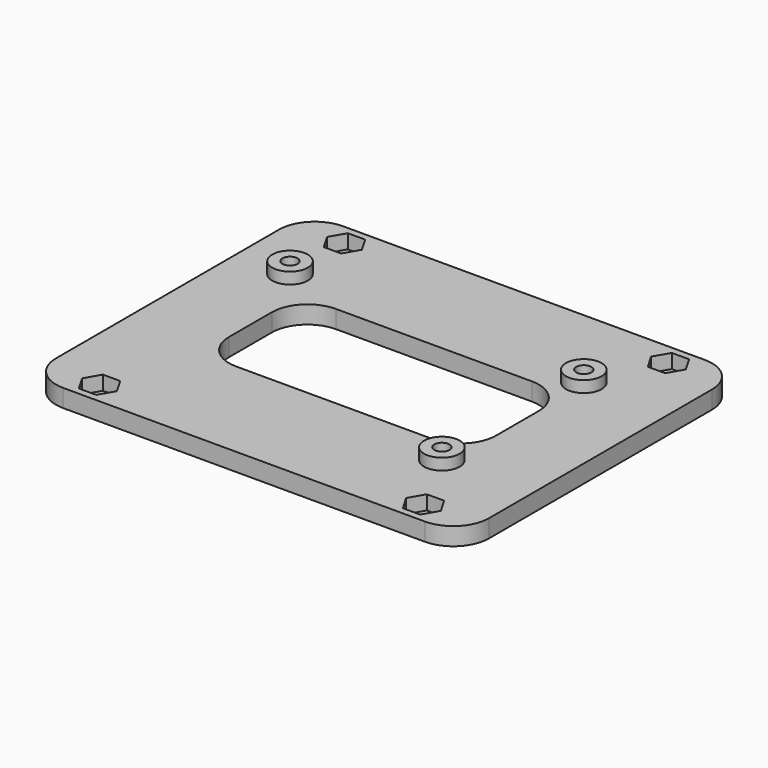
from build123d import *

# Parameters (mm, degrees)
F0_W         = 121.6
F0_H         = 78.3
F0_R         = 2.125
F1_DEPTH     = 5
F2_R         = 5
F2_R_2       = 2.125
F3_DEPTH     = 3.2
F5_DEPTH     = 4
F6_W         = 121.6
F6_H         = 10
F6_R         = 2.25
F7_DEPTH     = 5
F8_R         = 10
F9_T3_DEPTH  = 9.8067065447
F9_S4_R      = 2.125
F9_T5_DEPTH  = 7
F9_T8_DEPTH  = 9.8067065447
F9_S9_R      = 2.125
F9_T10_DEPTH = 6
F9_T13_DEPTH = 9.8067065447
F9_S14_R     = 2.125
F9_T15_DEPTH = 7
F9_T18_DEPTH = 9.8067065447
F9_S19_R     = 2.125
F9_T20_DEPTH = 7
F9_T23_DEPTH = 9.8067065447
F9_S24_R     = 2.125
F9_T25_DEPTH = 7
F9_T28_DEPTH = 9.8067065447
F9_S29_R     = 2.125
F9_T30_DEPTH = 6
F9_T33_DEPTH = 9.8067065447
F9_S34_R     = 2.125
F9_T35_DEPTH = 6
F9_T38_DEPTH = 9.8067065447
F9_S39_R     = 2.125
F9_T40_DEPTH = 7
F9_T43_DEPTH = 9.8067065447
F9_S44_R     = 2.125
F9_T45_DEPTH = 7
F9_T48_DEPTH = 9.8067065447
F9_S49_R     = 2.125
F9_T50_DEPTH = 7
F9_T53_DEPTH = 9.8067065447
F9_S54_R     = 2.125
F9_T55_DEPTH = 7
F9_T58_DEPTH = 9.8067065447
F9_S59_R     = 2.125
F9_T60_DEPTH = 6
F9_T63_DEPTH = 9.8067065447
F9_S64_R     = 2.125
F9_T65_DEPTH = 7
F9_T68_DEPTH = 9.8067065447
F9_S69_R     = 2.125
F9_T70_DEPTH = 6
F9_T73_DEPTH = 9.8067065447
F9_S74_R     = 2.125
F9_T75_DEPTH = 7
F9_T78_DEPTH = 9.8067065447
F9_S79_R     = 2.125
F9_T80_DEPTH = 7
F9_T83_DEPTH = 9.8067065447
F9_S84_R     = 2.125
F9_T85_DEPTH = 6
F9_T88_DEPTH = 9.8067065447
F9_S89_R     = 2.125
F9_T90_DEPTH = 7
F11_DEPTH    = 4


# Not quite as in the source:
# - a fillet or chamfer that OpenCascade refuses, or shapes differently, is made with other operations: its cross-section is extruded or revolved along the edge and cut away or added


with BuildPart() as f1:
    # F0 (on Top) → F1 (new body)
    with BuildSketch(Plane.XY):
        Rectangle(F0_W, F0_H)
        with Locations((35.5, -24.05)):
            Circle(F0_R, mode=Mode.SUBTRACT)
        with BuildLine():
            ThreePointArc((37.5, -7.5), (34.5710678119, -14.5710678119), (27.5, -17.5))
            Line((27.5, -17.5), (-27.5, -17.5))
            ThreePointArc((-27.5, -17.5), (-34.5710678119, -14.5710678119), (-37.5, -7.5))
            Line((-37.5, -7.5), (-37.5, 7.5))
            ThreePointArc((-37.5, 7.5), (-34.5710678119, 14.5710678119), (-27.5, 17.5))
            Line((-27.5, 17.5), (27.5, 17.5))
            ThreePointArc((27.5, 17.5), (34.5710678119, 14.5710678119), (37.5, 7.5))
            Line((37.5, 7.5), (37.5, -7.5))
        make_face(mode=Mode.SUBTRACT)
        with Locations((-45.72, 24.15)):
            Circle(F0_R, mode=Mode.SUBTRACT)
        with Locations((36.8, 24.15)):
            Circle(F0_R, mode=Mode.SUBTRACT)
    extrude(amount=F1_DEPTH)

    # F2 (on face) → F3 (join)
    with BuildSketch(Plane.XY.offset(5)):
        with Locations((-45.72, 24.15)):
            Circle(F2_R)
        with Locations((-45.72, 24.15)):
            Circle(F2_R_2, mode=Mode.SUBTRACT)
        with Locations((36.8, 24.15)):
            Circle(F2_R)
        with Locations((36.8, 24.15)):
            Circle(F2_R_2, mode=Mode.SUBTRACT)
        with Locations((35.5, -24.05)):
            Circle(F2_R)
        with Locations((35.5, -24.05)):
            Circle(F2_R_2, mode=Mode.SUBTRACT)
    extrude(amount=F3_DEPTH)

    # F4 (on face) → F5 (cut)
    with BuildSketch(Plane(origin=(0, 0, 0), x_dir=(1, 0, 0), z_dir=(0, 0, -1))):
        Polygon((-44.0312504626, -21.225), (-47.4087495374, -21.225), (-49.0974990748, -24.15), (-47.4087495374, -27.075), (-44.0312504626, -27.075), (-42.3425009252, -24.15), align=None)
        Polygon((38.4887495374, -21.225), (35.1112504626, -21.225), (33.4225009252, -24.15), (35.1112504626, -27.075), (38.4887495374, -27.075), (40.1774990748, -24.15), align=None)
        Polygon((33.8112504626, 21.125), (37.1887495374, 21.125), (38.8774990748, 24.05), (37.1887495374, 26.975), (33.8112504626, 26.975), (32.1225009252, 24.05), align=None)
    extrude(amount=-F5_DEPTH, mode=Mode.SUBTRACT)

    # F6 (on Top) → F7 (join)
    with BuildSketch(Plane.XY):
        with Locations((0, 44.15)):
            Rectangle(F6_W, F6_H)
        with Locations((-45.5, 43)):
            Circle(F6_R, mode=Mode.SUBTRACT)
        with Locations((45.5, 43)):
            Circle(F6_R, mode=Mode.SUBTRACT)
        with Locations((0, -44.15)):
            Rectangle(F6_W, F6_H)
        with Locations((-45.5, -43)):
            Circle(F6_R, mode=Mode.SUBTRACT)
        with Locations((45.5, -43)):
            Circle(F6_R, mode=Mode.SUBTRACT)
    extrude(amount=F7_DEPTH)

    # F8
    f8_edges = [f1.edges().sort_by_distance(p)[0] for p in [
        (-60.8, 49.15, 2.5),
        (60.8, 49.15, 2.5),
        (-60.8, -49.15, 2.5),
        (60.8, -49.15, 2.5),
    ]]
    fillet(f8_edges, radius=F8_R)

    # F9: chamfer of 1.25 on 18 edges, made by hand


with BuildPart() as f9_tool1:
    # F9_s2 → F9_t3 (new body)
    with BuildSketch(Plane(origin=(0.9127211557, 1.5808794147, 0), x_dir=(0, 0, 1), z_dir=(-0.5, -0.8660254038, 0))):
        Polygon((2.75, -45.6939018343), (4, -44.4439018343), (4, -45.6939018343), align=None)
    extrude(amount=F9_T3_DEPTH)

    # F9_s4 → F9_t5 (cut, symmetric)
    with BuildSketch(Plane.XY.offset(3.4)):
        with Locations((35.5, -24.05)):
            Circle(F9_S4_R)
    extrude(amount=F9_T5_DEPTH, both=True, mode=Mode.SUBTRACT)


with BuildPart() as f9_tool6:
    # F9_s7 → F9_t8 (new body)
    with BuildSketch(Plane.YZ.offset(40.4033532723)):
        Polygon((-26.975, 2.75), (-25.725, 4), (-26.975, 4), align=None)
    extrude(amount=-F9_T8_DEPTH)

    # F9_s9 → F9_t10 (cut, symmetric)
    with BuildSketch(Plane.XY.offset(3.4)):
        with Locations((35.5, -24.05)):
            Circle(F9_S9_R)
    extrude(amount=F9_T10_DEPTH, both=True, mode=Mode.SUBTRACT)


with BuildPart() as f9_tool11:
    # F9_s12 → F9_t13 (new body)
    with BuildSketch(Plane(origin=(21.7406321167, -37.6558794147, 0), x_dir=(0, 0, 1), z_dir=(-0.5, 0.8660254038, 0))):
        Polygon((2.75, 15.7939018343), (4, 17.0439018343), (4, 15.7939018343), align=None)
    extrude(amount=F9_T13_DEPTH)

    # F9_s14 → F9_t15 (cut, symmetric)
    with BuildSketch(Plane.XY.offset(3.4)):
        with Locations((35.5, -24.05)):
            Circle(F9_S14_R)
    extrude(amount=F9_T15_DEPTH, both=True, mode=Mode.SUBTRACT)


with BuildPart() as f9_tool16:
    # F9_s17 → F9_t18 (new body)
    with BuildSketch(Plane(origin=(-3.9906321167, -6.9119775804, 0), x_dir=(0, 0, 1), z_dir=(0.5, 0.8660254038, 0))):
        Polygon((2.75, 39.8439018343), (4, 41.0939018343), (4, 39.8439018343), align=None)
    extrude(amount=F9_T18_DEPTH)

    # F9_s19 → F9_t20 (cut, symmetric)
    with BuildSketch(Plane.XY.offset(3.4)):
        with Locations((35.5, -24.05)):
            Circle(F9_S19_R)
    extrude(amount=F9_T20_DEPTH, both=True, mode=Mode.SUBTRACT)


with BuildPart() as f9_tool21:
    # F9_s22 → F9_t23 (new body)
    with BuildSketch(Plane(origin=(16.8372788443, -29.1630224196, 0), x_dir=(0, 0, 1), z_dir=(0.5, -0.8660254038, 0))):
        Polygon((2.75, -21.6439018343), (4, -20.3939018343), (4, -21.6439018343), align=None)
    extrude(amount=F9_T23_DEPTH)

    # F9_s24 → F9_t25 (cut, symmetric)
    with BuildSketch(Plane.XY.offset(3.4)):
        with Locations((35.5, -24.05)):
            Circle(F9_S24_R)
    extrude(amount=F9_T25_DEPTH, both=True, mode=Mode.SUBTRACT)


with BuildPart() as f9_tool26:
    # F9_s27 → F9_t28 (new body)
    with BuildSketch(Plane.YZ.offset(30.5966467277)):
        Polygon((-21.125, 2.75), (-22.375, 4), (-21.125, 4), align=None)
    extrude(amount=F9_T28_DEPTH)

    # F9_s29 → F9_t30 (cut, symmetric)
    with BuildSketch(Plane.XY.offset(3.4)):
        with Locations((35.5, -24.05)):
            Circle(F9_S29_R)
    extrude(amount=F9_T30_DEPTH, both=True, mode=Mode.SUBTRACT)


with BuildPart() as f9_tool31:
    # F9_s32 → F9_t33 (new body)
    with BuildSketch(Plane.YZ.offset(41.7033532723)):
        Polygon((21.225, 2.75), (22.475, 4), (21.225, 4), align=None)
    extrude(amount=-F9_T33_DEPTH)

    # F9_s34 → F9_t35 (cut, symmetric)
    with BuildSketch(Plane.XY.offset(3.4)):
        with Locations((36.8, 24.15)):
            Circle(F9_S34_R)
    extrude(amount=F9_T35_DEPTH, both=True, mode=Mode.SUBTRACT)


with BuildPart() as f9_tool36:
    # F9_s37 → F9_t38 (new body)
    with BuildSketch(Plane(origin=(1.1944198855, -2.0687959272, 0), x_dir=(0, 0, 1), z_dir=(-0.5, 0.8660254038, 0))):
        Polygon((2.75, 41.0197348593), (4, 42.2697348593), (4, 41.0197348593), align=None)
    extrude(amount=F9_T38_DEPTH)

    # F9_s39 → F9_t40 (cut, symmetric)
    with BuildSketch(Plane.XY.offset(3.4)):
        with Locations((36.8, 24.15)):
            Circle(F9_S39_R)
    extrude(amount=F9_T40_DEPTH, both=True, mode=Mode.SUBTRACT)


with BuildPart() as f9_tool41:
    # F9_s42 → F9_t43 (new body)
    with BuildSketch(Plane(origin=(17.2055801145, 29.8009389321, 0), x_dir=(0, 0, 1), z_dir=(0.5, 0.8660254038, 0))):
        Polygon((2.75, 16.8697348593), (4, 18.1197348593), (4, 16.8697348593), align=None)
    extrude(amount=F9_T43_DEPTH)

    # F9_s44 → F9_t45 (cut, symmetric)
    with BuildSketch(Plane.XY.offset(3.4)):
        with Locations((36.8, 24.15)):
            Circle(F9_S44_R)
    extrude(amount=F9_T45_DEPTH, both=True, mode=Mode.SUBTRACT)


with BuildPart() as f9_tool46:
    # F9_s47 → F9_t48 (new body)
    with BuildSketch(Plane(origin=(22.1089333869, 38.2937959272, 0), x_dir=(0, 0, 1), z_dir=(-0.5, -0.8660254038, 0))):
        Polygon((2.75, -22.7197348593), (4, -21.4697348593), (4, -22.7197348593), align=None)
    extrude(amount=F9_T48_DEPTH)

    # F9_s49 → F9_t50 (cut, symmetric)
    with BuildSketch(Plane.XY.offset(3.4)):
        with Locations((36.8, 24.15)):
            Circle(F9_S49_R)
    extrude(amount=F9_T50_DEPTH, both=True, mode=Mode.SUBTRACT)


with BuildPart() as f9_tool51:
    # F9_s52 → F9_t53 (new body)
    with BuildSketch(Plane(origin=(-3.7089333869, 6.4240610679, 0), x_dir=(0, 0, 1), z_dir=(0.5, -0.8660254038, 0))):
        Polygon((2.75, -46.8697348593), (4, -45.6197348593), (4, -46.8697348593), align=None)
    extrude(amount=F9_T53_DEPTH)

    # F9_s54 → F9_t55 (cut, symmetric)
    with BuildSketch(Plane.XY.offset(3.4)):
        with Locations((36.8, 24.15)):
            Circle(F9_S54_R)
    extrude(amount=F9_T55_DEPTH, both=True, mode=Mode.SUBTRACT)


with BuildPart() as f9_tool56:
    # F9_s57 → F9_t58 (new body)
    with BuildSketch(Plane.YZ.offset(31.8966467277)):
        Polygon((27.075, 2.75), (25.825, 4), (27.075, 4), align=None)
    extrude(amount=F9_T58_DEPTH)

    # F9_s59 → F9_t60 (cut, symmetric)
    with BuildSketch(Plane.XY.offset(3.4)):
        with Locations((36.8, 24.15)):
            Circle(F9_S59_R)
    extrude(amount=F9_T60_DEPTH, both=True, mode=Mode.SUBTRACT)


with BuildPart() as f9_tool61:
    # F9_s62 → F9_t63 (new body)
    with BuildSketch(Plane(origin=(-24.3389333869, 42.1562692281, 0), x_dir=(0, 0, 1), z_dir=(0.5, -0.8660254038, 0))):
        Polygon((2.75, 24.594681461), (4, 25.844681461), (4, 24.594681461), align=None)
    extrude(amount=F9_T63_DEPTH)

    # F9_s64 → F9_t65 (cut, symmetric)
    with BuildSketch(Plane.XY.offset(3.4)):
        with Locations((-45.72, 24.15)):
            Circle(F9_S64_R)
    extrude(amount=F9_T65_DEPTH, both=True, mode=Mode.SUBTRACT)


with BuildPart() as f9_tool66:
    # F9_s67 → F9_t68 (new body)
    with BuildSketch(Plane.YZ.offset(-50.6233532723)):
        Polygon((27.075, 2.75), (25.825, 4), (27.075, 4), align=None)
    extrude(amount=F9_T68_DEPTH)

    # F9_s69 → F9_t70 (cut, symmetric)
    with BuildSketch(Plane.XY.offset(3.4)):
        with Locations((-45.72, 24.15)):
            Circle(F9_S69_R)
    extrude(amount=F9_T70_DEPTH, both=True, mode=Mode.SUBTRACT)


with BuildPart() as f9_tool71:
    # F9_s72 → F9_t73 (new body)
    with BuildSketch(Plane(origin=(-3.4244198855, -5.9312692281, 0), x_dir=(0, 0, 1), z_dir=(0.5, 0.8660254038, 0))):
        Polygon((2.75, -54.594681461), (4, -53.344681461), (4, -54.594681461), align=None)
    extrude(amount=F9_T73_DEPTH)

    # F9_s74 → F9_t75 (cut, symmetric)
    with BuildSketch(Plane.XY.offset(3.4)):
        with Locations((-45.72, 24.15)):
            Circle(F9_S74_R)
    extrude(amount=F9_T75_DEPTH, both=True, mode=Mode.SUBTRACT)


with BuildPart() as f9_tool76:
    # F9_s77 → F9_t78 (new body)
    with BuildSketch(Plane(origin=(1.4789333869, 2.5615877671, 0), x_dir=(0, 0, 1), z_dir=(-0.5, -0.8660254038, 0))):
        Polygon((2.75, 48.744681461), (4, 49.994681461), (4, 48.744681461), align=None)
    extrude(amount=F9_T78_DEPTH)

    # F9_s79 → F9_t80 (cut, symmetric)
    with BuildSketch(Plane.XY.offset(3.4)):
        with Locations((-45.72, 24.15)):
            Circle(F9_S79_R)
    extrude(amount=F9_T80_DEPTH, both=True, mode=Mode.SUBTRACT)


with BuildPart() as f9_tool81:
    # F9_s82 → F9_t83 (new body)
    with BuildSketch(Plane.YZ.offset(-40.8166467277)):
        Polygon((21.225, 2.75), (22.475, 4), (21.225, 4), align=None)
    extrude(amount=-F9_T83_DEPTH)

    # F9_s84 → F9_t85 (cut, symmetric)
    with BuildSketch(Plane.XY.offset(3.4)):
        with Locations((-45.72, 24.15)):
            Circle(F9_S84_R)
    extrude(amount=F9_T85_DEPTH, both=True, mode=Mode.SUBTRACT)


with BuildPart() as f9_tool86:
    # F9_s87 → F9_t88 (new body)
    with BuildSketch(Plane(origin=(-19.4355801145, 33.6634122329, 0), x_dir=(0, 0, 1), z_dir=(-0.5, 0.8660254038, 0))):
        Polygon((2.75, -30.444681461), (4, -29.194681461), (4, -30.444681461), align=None)
    extrude(amount=F9_T88_DEPTH)

    # F9_s89 → F9_t90 (cut, symmetric)
    with BuildSketch(Plane.XY.offset(3.4)):
        with Locations((-45.72, 24.15)):
            Circle(F9_S89_R)
    extrude(amount=F9_T90_DEPTH, both=True, mode=Mode.SUBTRACT)


with BuildPart() as f1_1:
    add(f1.part)

    # F9_t91: union F9_tool1, F9_tool6, F9_tool11, F9_tool16, F9_tool21, F9_tool26, F9_tool31, F9_tool36, F9_tool41, F9_tool46, F9_tool51, F9_tool56, F9_tool61, F9_tool66, F9_tool71, F9_tool76, F9_tool81, F9_tool86
    add([f9_tool1.part, f9_tool6.part, f9_tool11.part, f9_tool16.part, f9_tool21.part, f9_tool26.part, f9_tool31.part, f9_tool36.part, f9_tool41.part, f9_tool46.part, f9_tool51.part, f9_tool56.part, f9_tool61.part, f9_tool66.part, f9_tool71.part, f9_tool76.part, f9_tool81.part, f9_tool86.part])

    # F10 (on face) → F11 (cut)
    with BuildSketch(Plane.XY.offset(5)):
        Polygon((-43.0606951127, 47.225), (-47.9393048873, 47.225), (-50.3786097747, 43), (-47.9393048873, 38.775), (-43.0606951127, 38.775), (-40.6213902253, 43), align=None)
        Polygon((47.9393048873, 38.775), (50.3786097747, 43), (47.9393048873, 47.225), (43.0606951127, 47.225), (40.6213902253, 43), (43.0606951127, 38.775), align=None)
        Polygon((50.3786097747, -43), (47.9393048873, -38.775), (43.0606951127, -38.775), (40.6213902253, -43), (43.0606951127, -47.225), (47.9393048873, -47.225), align=None)
        Polygon((-50.3786097747, -43), (-47.9393048873, -47.225), (-43.0606951127, -47.225), (-40.6213902253, -43), (-43.0606951127, -38.775), (-47.9393048873, -38.775), align=None)
    extrude(amount=-F11_DEPTH, mode=Mode.SUBTRACT)


solid = f1_1.part
